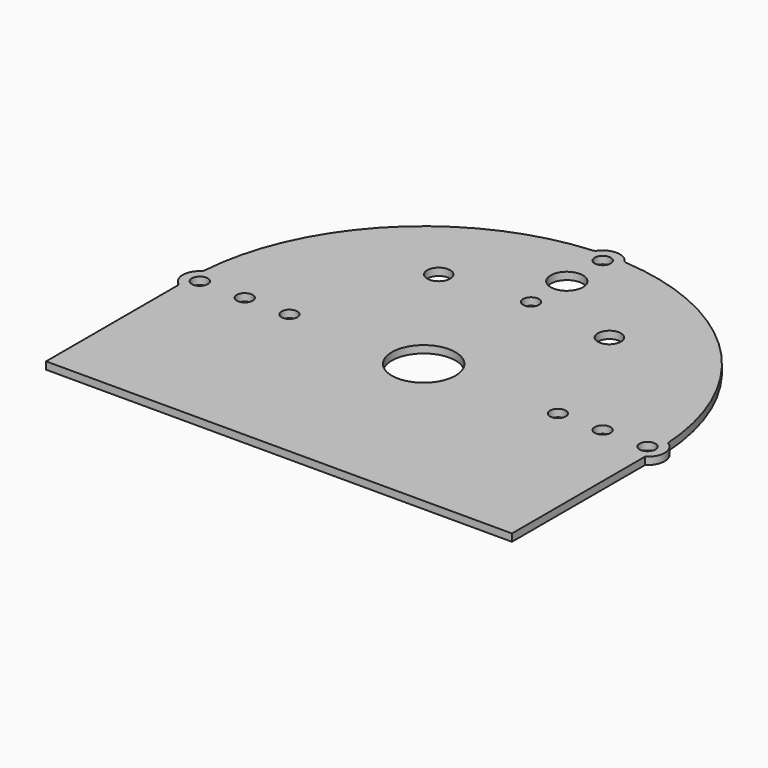
from build123d import *

# Parameters (mm, degrees)
F0_R     = 8.631475
F0_R_2   = 8.6
F0_R_3   = 34.5
F0_R_4   = 12.5
F0_R_5   = 17.5
F1_DEPTH = 8


# Not quite as in the source:
# - ends of sketch curves that miss each other by under 0.0002 mm in the source are joined


with BuildPart() as f1:
    # F0 (on Top) → F1 (new body)
    with BuildSketch(Plane.XY):
        with BuildLine():
            ThreePointArc((18.476772036, 219.2230704901), (16.4501234267, 219.819241628), (14.8505619493, 221.1991429618))
            ThreePointArc((14.8505619493, 221.1991429618), (3.011e-07, 228.6), (-14.8505617308, 221.1991435511))
            ThreePointArc((-14.8505617308, 221.1991435511), (-16.4501227245, 219.8192420107), (-18.4767710413, 219.2230705631))
            ThreePointArc((-18.4767710413, 219.2230705631), (-178.5444622496, 145.9444622496), (-251.8230706896, -14.1232289494))
            ThreePointArc((-251.8230706896, -14.1232289494), (-252.4192420107, -16.1498772755), (-253.7991434425, -17.7494384132))
            ThreePointArc((-253.7991434425, -17.7494384132), (-261.1967885287, -32.2543753223), (-254.343219804, -47.0241737592))
            ThreePointArc((-254.343219804, -47.0241737592), (-252.9842553662, -48.7550030017), (-252.5, -50.90164))
            Line((-252.5, -50.90164), (-252.5, -228.6))
            Line((-252.5, -228.6), (252.5, -228.6))
            Line((252.5, -228.6), (252.5, -48.346429))
            ThreePointArc((252.5, -48.346429), (261.1975992169, -32.3011633084), (251.9889742877, -16.5436255081))
            ThreePointArc((251.9889742877, -16.5436255081), (179.4001497018, 145.0846540559), (18.476772036, 219.2230704901))
        make_face()
        with Locations((-242.6, -32.6)):
            Circle(F0_R, mode=Mode.SUBTRACT)
        with Locations((-194, -32.6)):
            Circle(F0_R_2, mode=Mode.SUBTRACT)
        with Locations((-145.5, -32.6)):
            Circle(F0_R_2, mode=Mode.SUBTRACT)
        with Locations((0, -32.6)):
            Circle(F0_R_3, mode=Mode.SUBTRACT)
        with Locations((145.5, -32.6)):
            Circle(F0_R_2, mode=Mode.SUBTRACT)
        with Locations((194, -32.6)):
            Circle(F0_R_2, mode=Mode.SUBTRACT)
        with Locations((242.6, -32.6)):
            Circle(F0_R, mode=Mode.SUBTRACT)
        with Locations((-92.5, 103.4)):
            Circle(F0_R_4, mode=Mode.SUBTRACT)
        with Locations((0, 112.9)):
            Circle(F0_R_2, mode=Mode.SUBTRACT)
        with Locations((92.5, 103.4)):
            Circle(F0_R_4, mode=Mode.SUBTRACT)
        with Locations((0, 161.4)):
            Circle(F0_R_5, mode=Mode.SUBTRACT)
        with Locations((0, 210)):
            Circle(F0_R, mode=Mode.SUBTRACT)
    extrude(amount=F1_DEPTH)


solid = f1.part
